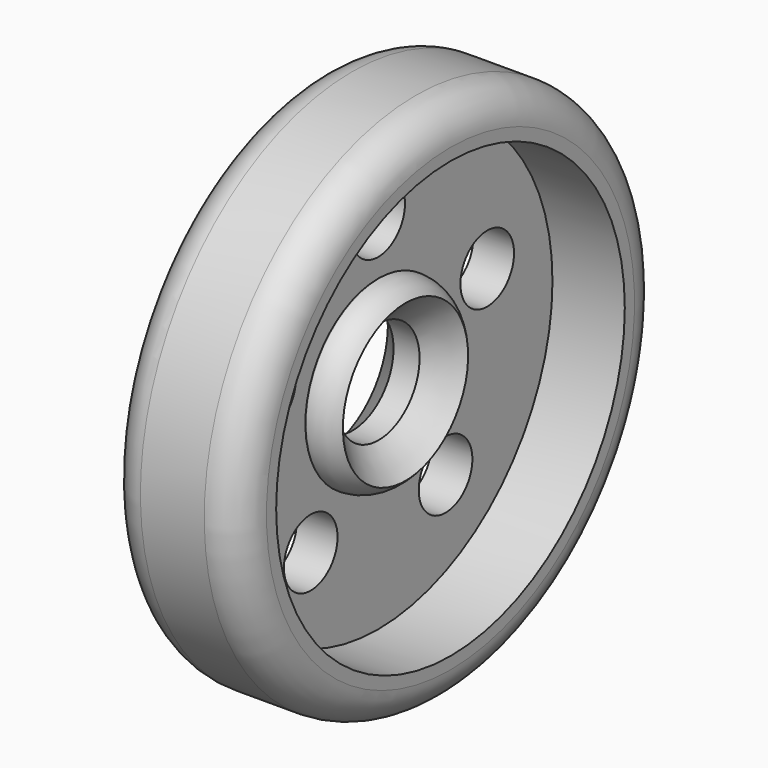
from build123d import *

# Parameters (mm, degrees)
F2_R     = 4.7917393222
F3_DEPTH = 25


# Not quite as in the source:
# - a fillet or chamfer that OpenCascade refuses, or shapes differently, is made with other operations: its cross-section is extruded or revolved along the edge and cut away or added


with BuildPart() as f1:
    # F0 (on Front) → F1 (revolve)
    with BuildSketch(Plane.XZ):
        Polygon((0, 12.9990037531), (0, 7.3299529031), (13.7201668695, 7.3299529031), (13.7201668695, 12.9990037531), (8.6628543213, 12.9990037531), (8.6628543213, 31.1359390616), (18.9999677241, 31.1359390616), (18.9999677241, 37.8080755472), (0, 37.8080755472), (0, 31.1359390616), (2.8364819009, 31.1359390616), (2.8364819009, 12.9990037531), align=None)
    revolve(axis=Axis((6.8600834347, 0, 0), (1, 0, 0)))

    # F2 (on face) → F3 (cut)
    with BuildSketch(Plane.YZ.offset(8.6628543213)):
        with Locations((-19.483606852, 6.3306076199)):
            Circle(F2_R)
        with Locations((0, 20.4862765968)):
            Circle(F2_R)
        with Locations((19.483606852, 6.3306076199)):
            Circle(F2_R)
        with Locations((12.041531258, -16.5737459183)):
            Circle(F2_R)
        with Locations((-12.041531258, -16.5737459183)):
            Circle(F2_R)
    extrude(amount=-F3_DEPTH, mode=Mode.SUBTRACT)

    # F4: fillet of radius 5 on 4 edges, made by hand

    # F4_s1 → F4_t2 (revolve, cut)
    with BuildSketch(Plane.XZ):
        with BuildLine():
            ThreePointArc((-0.0004, 32.8071098618), (1.4644660941, 36.3436094532), (5.0009656854, 37.8084755472))
            Line((5.0009656854, 37.8084755472), (5.0009656854, 38.3086121158))
            ThreePointArc((5.0009656854, 38.3086121158), (2.5004828427, 38.3082121158), (0, 38.3082121158))
            Line((0, 38.3082121158), (-0.5001365685, 37.8080755472))
            ThreePointArc((-0.5001365685, 37.8080755472), (-0.5001365685, 35.3075927045), (-0.5005365685, 32.8071098618))
            Line((-0.5005365685, 32.8071098618), (-0.0004, 32.8071098618))
        make_face()
    revolve(axis=Axis((0, 0, 0), (1, 0, 0)), mode=Mode.SUBTRACT)

    # F4_s3 → F4_t4 (revolve, cut)
    with BuildSketch(Plane.XZ):
        with BuildLine():
            ThreePointArc((13.9990020387, 37.8084755472), (17.53550163, 36.3436094532), (19.0003677241, 32.8071098618))
            Line((19.0003677241, 32.8071098618), (19.5005042926, 32.8071098618))
            ThreePointArc((19.5005042926, 32.8071098618), (19.5001042926, 35.3075927045), (19.5001042926, 37.8080755472))
            Line((19.5001042926, 37.8080755472), (18.9999677241, 38.3082121158))
            ThreePointArc((18.9999677241, 38.3082121158), (16.4994848814, 38.3082121158), (13.9990020387, 38.3086121158))
            Line((13.9990020387, 38.3086121158), (13.9990020387, 37.8084755472))
        make_face()
    revolve(axis=Axis((18.9999677241, 0, 0), (1, 0, 0)), mode=Mode.SUBTRACT)

    # F4_s5 → F4_t6 (revolve, cut)
    with BuildSketch(Plane.XZ):
        with BuildLine():
            ThreePointArc((-0.0004, 8.490714972), (0.7677695224, 11.1541167376), (2.8363087756, 12.9993643465))
            Line((2.8363087756, 12.9993643465), (2.6198430846, 13.450229284))
            ThreePointArc((2.6198430846, 13.450229284), (1.4181543878, 13.4991403216), (0, 13.4991403216))
            Line((0, 13.4991403216), (-0.5001365685, 12.9990037531))
            ThreePointArc((-0.5001365685, 12.9990037531), (-0.5001365685, 10.7448593625), (-0.5005365685, 8.490714972))
            Line((-0.5005365685, 8.490714972), (-0.0004, 8.490714972))
        make_face()
    revolve(axis=Axis((0, 0, 0), (1, 0, 0)), mode=Mode.SUBTRACT)

    # F4_s7 → F4_t8 (revolve, cut)
    with BuildSketch(Plane.XZ):
        with BuildLine():
            ThreePointArc((13.7205668695, 7.9980380676), (12.2557007754, 11.534537659), (8.719201184, 12.9994037531))
            Line((8.719201184, 12.9994037531), (8.719201184, 13.4995403216))
            ThreePointArc((8.719201184, 13.4995403216), (11.2196840267, 13.4991403216), (13.7201668695, 13.4991403216))
            Line((13.7201668695, 13.4991403216), (14.220303438, 12.9990037531))
            ThreePointArc((14.220303438, 12.9990037531), (14.220303438, 10.4985209104), (14.220703438, 7.9980380676))
            Line((14.220703438, 7.9980380676), (13.7205668695, 7.9980380676))
        make_face()
    revolve(axis=Axis((13.7201668695, 0, 0), (1, 0, 0)), mode=Mode.SUBTRACT)

    # F5: chamfer of 5 on 3 edges, made by hand

    # F5_s1 → F5_t2 (revolve, cut)
    with BuildSketch(Plane.XZ):
        Polygon((0, 12.3299529031), (5, 7.3299529031), (0, 7.3299529031), align=None)
    revolve(axis=Axis((0, 0, 0), (1, 0, 0)), mode=Mode.SUBTRACT)

    # F5_s3 → F5_t4 (revolve, cut)
    with BuildSketch(Plane.XZ):
        Polygon((8.7201668695, 7.3299529031), (13.7201668695, 12.3299529031), (13.7201668695, 7.3299529031), align=None)
    revolve(axis=Axis((13.7201668695, 0, 0), (1, 0, 0)), mode=Mode.SUBTRACT)


solid = f1.part
